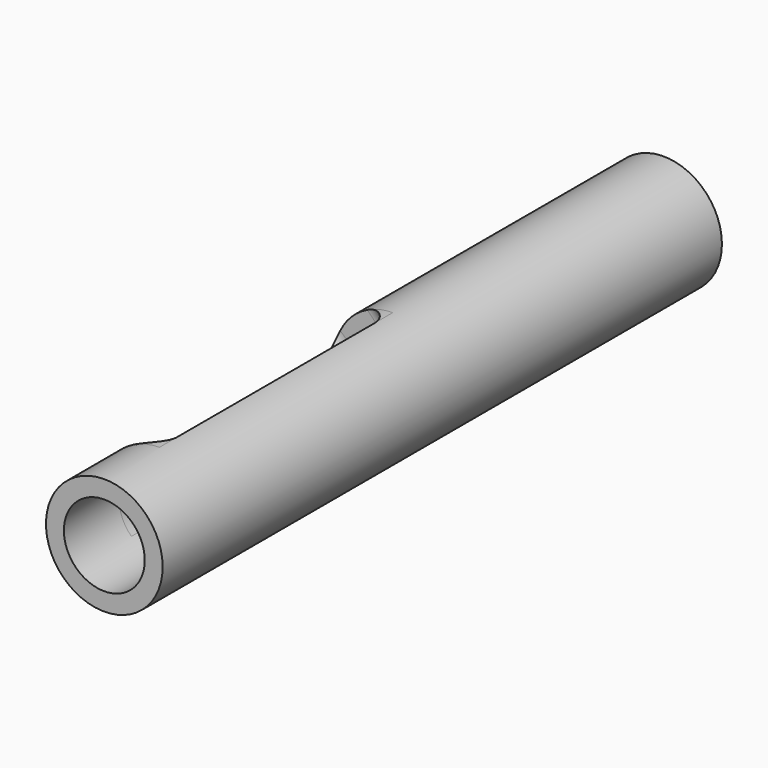
from build123d import *

# Parameters (mm, degrees)
F0_R         = 16.5608
F0_R_2       = 11.4808
F1_DEPTH     = 198.4502
F4_DEPTH     = 82.804
F5_T4_DEPTH  = 43.6852975665
F5_S5_R      = 16.5608
F5_T6_DEPTH  = 27
F5_S7_R      = 11.4808
F5_T8_DEPTH  = 27
F5_T12_DEPTH = 43.6852975665
F5_S13_R     = 16.5608
F5_T14_DEPTH = 27
F5_S15_R     = 11.4808
F5_T16_DEPTH = 27
F5_T20_DEPTH = 43.6852975665
F5_S21_R     = 16.5608
F5_T22_DEPTH = 27
F5_S23_R     = 11.4808
F5_T24_DEPTH = 27
F5_T28_DEPTH = 43.6852975665
F5_S29_R     = 16.5608
F5_T30_DEPTH = 27
F5_S31_R     = 11.4808
F5_T32_DEPTH = 27


# Not quite as in the source:
# - a fillet or chamfer that OpenCascade refuses, or shapes differently, is made with other operations: its cross-section is extruded or revolved along the edge and cut away or added


with BuildPart() as f1:
    # F0 (on Front) → F1 (new body)
    with BuildSketch(Plane.XZ):
        Circle(F0_R)
        Circle(F0_R_2, mode=Mode.SUBTRACT)
    extrude(amount=F1_DEPTH)

    # F3 (on offset) → F4 (cut)
    with BuildSketch(Plane(origin=(0, -96.0882, 0), x_dir=(-1, 0, 0), z_dir=(0, 1, 0))):
        with BuildLine():
            Line((7.9590822086, -8.2741633436), (16.5608, 0))
            ThreePointArc((16.5608, 0), (11.7102539819, 11.7102539819), (0, 16.5608))
            Line((0, 16.5608), (-8.2741633436, 7.9590822086))
            Line((-8.2741633436, 7.9590822086), (7.9590822086, -8.2741633436))
        make_face()
    extrude(amount=-F4_DEPTH, mode=Mode.SUBTRACT)

    # F5: fillet of radius 6.35 on 4 edges, made by hand


with BuildPart() as f5_tool2:
    # F5_s3 → F5_t4 (new body)
    with BuildSketch(Plane(origin=(-19.2795314418, 0, 20.0427622378), x_dir=(0, 1, 0), z_dir=(0.6932515337, 0, -0.7206957132))):
        with BuildLine():
            ThreePointArc((-102.4382, 11.4808), (-97.9480719395, 9.6209280605), (-96.0882, 5.1308))
            Line((-96.0882, 5.1308), (-96.0882, 11.4808))
            Line((-96.0882, 11.4808), (-102.4382, 11.4808))
        make_face()
    extrude(amount=F5_T4_DEPTH)

    # F5_s5 → F5_t6 (intersect, symmetric)
    with BuildSketch(Plane.XZ.offset(99.3)):
        Circle(F5_S5_R)
    extrude(amount=F5_T6_DEPTH, both=True, mode=Mode.INTERSECT)

    # F5_s7 → F5_t8 (cut, symmetric)
    with BuildSketch(Plane.XZ.offset(99.3)):
        Circle(F5_S7_R)
    extrude(amount=F5_T8_DEPTH, both=True, mode=Mode.SUBTRACT)


with BuildPart() as f1_1:
    add(f1.part)

    # F5_t1: union F5_tool2
    add(f5_tool2.part)


with BuildPart() as f5_tool10:
    # F5_s11 → F5_t12 (new body)
    with BuildSketch(Plane(origin=(11.4410444464, 0, -11.0053680982), x_dir=(0, 1, 0), z_dir=(-0.7206957132, 0, 0.6932515337))):
        with BuildLine():
            ThreePointArc((-102.4382, 11.4808), (-97.9480719395, 9.6209280605), (-96.0882, 5.1308))
            Line((-96.0882, 5.1308), (-96.0882, 11.4808))
            Line((-96.0882, 11.4808), (-102.4382, 11.4808))
        make_face()
    extrude(amount=F5_T12_DEPTH)

    # F5_s13 → F5_t14 (intersect, symmetric)
    with BuildSketch(Plane.XZ.offset(99.3)):
        Circle(F5_S13_R)
    extrude(amount=F5_T14_DEPTH, both=True, mode=Mode.INTERSECT)

    # F5_s15 → F5_t16 (cut, symmetric)
    with BuildSketch(Plane.XZ.offset(99.3)):
        Circle(F5_S15_R)
    extrude(amount=F5_T16_DEPTH, both=True, mode=Mode.SUBTRACT)


with BuildPart() as f1_2:
    add(f1_1.part)

    # F5_t9: union F5_tool10
    add(f5_tool10.part)


with BuildPart() as f5_tool18:
    # F5_s19 → F5_t20 (new body)
    with BuildSketch(Plane(origin=(-19.2795314418, 0, 20.0427622378), x_dir=(0, 1, 0), z_dir=(0.6932515337, 0, -0.7206957132))):
        with BuildLine():
            ThreePointArc((-172.5422, 11.4808), (-177.0323280605, 9.6209280605), (-178.8922, 5.1308))
            Line((-178.8922, 5.1308), (-178.8922, 11.4808))
            Line((-178.8922, 11.4808), (-172.5422, 11.4808))
        make_face()
    extrude(amount=F5_T20_DEPTH)

    # F5_s21 → F5_t22 (intersect, symmetric)
    with BuildSketch(Plane.XZ.offset(175.7)):
        Circle(F5_S21_R)
    extrude(amount=F5_T22_DEPTH, both=True, mode=Mode.INTERSECT)

    # F5_s23 → F5_t24 (cut, symmetric)
    with BuildSketch(Plane.XZ.offset(175.7)):
        Circle(F5_S23_R)
    extrude(amount=F5_T24_DEPTH, both=True, mode=Mode.SUBTRACT)


with BuildPart() as f1_3:
    add(f1_2.part)

    # F5_t17: union F5_tool18
    add(f5_tool18.part)


with BuildPart() as f5_tool26:
    # F5_s27 → F5_t28 (new body)
    with BuildSketch(Plane(origin=(11.4410444464, 0, -11.0053680982), x_dir=(0, 1, 0), z_dir=(-0.7206957132, 0, 0.6932515337))):
        with BuildLine():
            ThreePointArc((-178.8922, 5.1308), (-177.0323280605, 9.6209280605), (-172.5422, 11.4808))
            Line((-172.5422, 11.4808), (-178.8922, 11.4808))
            Line((-178.8922, 11.4808), (-178.8922, 5.1308))
        make_face()
    extrude(amount=F5_T28_DEPTH)

    # F5_s29 → F5_t30 (intersect, symmetric)
    with BuildSketch(Plane.XZ.offset(175.7)):
        Circle(F5_S29_R)
    extrude(amount=F5_T30_DEPTH, both=True, mode=Mode.INTERSECT)

    # F5_s31 → F5_t32 (cut, symmetric)
    with BuildSketch(Plane.XZ.offset(175.7)):
        Circle(F5_S31_R)
    extrude(amount=F5_T32_DEPTH, both=True, mode=Mode.SUBTRACT)


with BuildPart() as f1_4:
    add(f1_3.part)

    # F5_t25: union F5_tool26
    add(f5_tool26.part)


solid = f1_4.part
